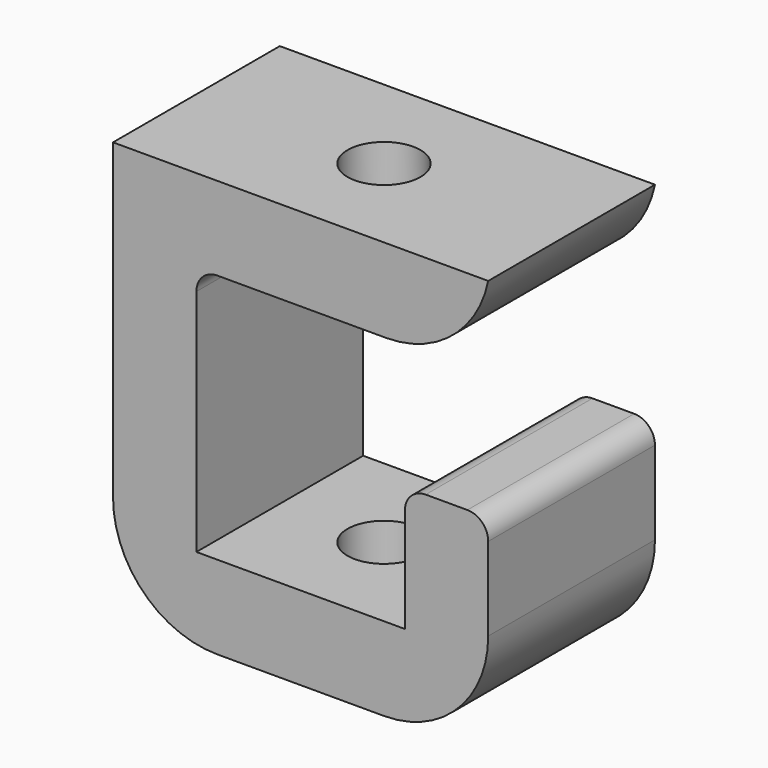
from build123d import *

# Parameters (mm, degrees)
F1_DEPTH    = 10
F2_T1_DEPTH = 34.4948974279
F2_T3_DEPTH = 35
F3_R        = 1
F4_R        = 1.75
F5_DEPTH    = 20.001
F6_SIZE     = 2


# Not quite as in the source:
# - a fillet or chamfer that OpenCascade refuses, or shapes differently, is made with other operations: its cross-section is extruded or revolved along the edge and cut away or added


with BuildPart() as f1:
    # F0 (on Front) → F1 (new body)
    with BuildSketch(Plane.XZ):
        Polygon((-18.6188016892, 16), (-18.6188016892, 20), (-36.6188016892, 20), (-36.6188016892, 0), (-18.6188016892, 0), (-18.6188016892, 10), (-22.6188016892, 10), (-22.6188016892, 4), (-32.6188016892, 4), (-32.6188016892, 16), align=None)
    extrude(amount=F1_DEPTH)

    # F2: fillet of radius 5 on 3 edges, made by hand

    # F2_s2 → F2_t1 (cut)
    with BuildSketch(Plane.XZ.offset(-12.2474487139)):
        with BuildLine():
            ThreePointArc((-23.5177811747, 16), (-20.3555035146, 17.1270166538), (-18.6188016892, 20))
            Line((-18.6188016892, 20), (-18.6188016892, 16))
            Line((-18.6188016892, 16), (-23.5177811747, 16))
        make_face()
    extrude(amount=F2_T1_DEPTH, mode=Mode.SUBTRACT)

    # F2_s4 → F2_t3 (cut)
    with BuildSketch(Plane.XZ.offset(-12.5)):
        with BuildLine():
            ThreePointArc((-18.6188016892, 5), (-20.0832677832, 1.4644660941), (-23.6188016892, 0))
            Line((-23.6188016892, 0), (-18.6188016892, 0))
            Line((-18.6188016892, 0), (-18.6188016892, 5))
        make_face()
        with BuildLine():
            ThreePointArc((-36.6188016892, 5), (-35.1543355951, 1.4644660941), (-31.6188016892, 0))
            Line((-31.6188016892, 0), (-36.6188016892, 0))
            Line((-36.6188016892, 0), (-36.6188016892, 5))
        make_face()
    extrude(amount=F2_T3_DEPTH, mode=Mode.SUBTRACT)

    # F3
    f3_edges = [f1.edges().sort_by_distance(p)[0] for p in [
        (-18.618802, -5, 10),
        (-22.618802, -5, 10),
        (-32.618802, -5, 16),
    ]]
    fillet(f3_edges, radius=F3_R)

    # F4 (on face) → F5 (cut, through all)
    with BuildSketch(Plane.XY.offset(20)):
        with Locations((-27.6188016892, -5)):
            Circle(F4_R)
    extrude(amount=-F5_DEPTH, mode=Mode.SUBTRACT)

    # F6
    f6_edges = [f1.edges().sort_by_distance(p)[0] for p in [
        (-29.368802, -5, 16),
    ]]
    chamfer(f6_edges, length=F6_SIZE)


solid = f1.part
